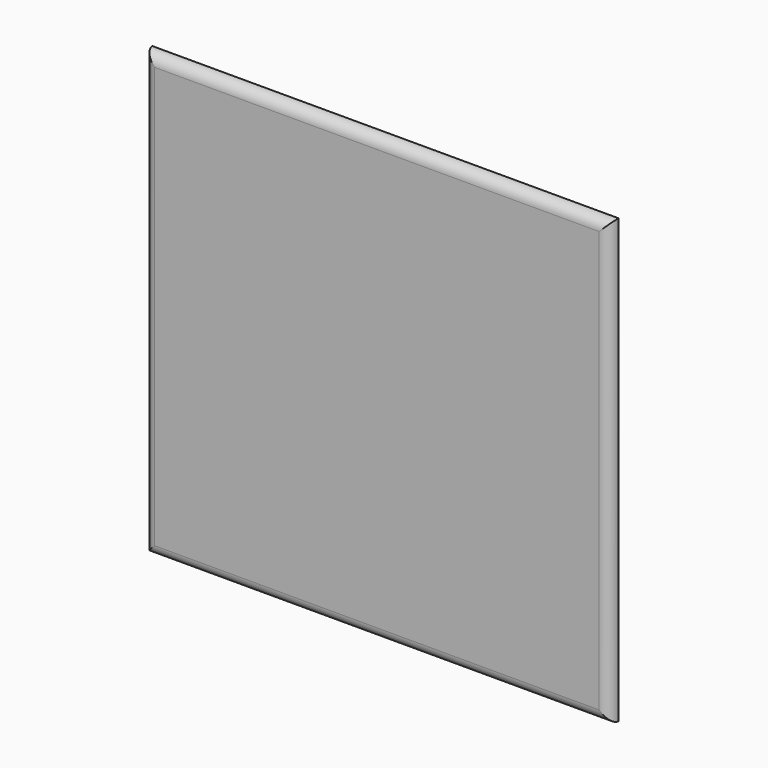
from build123d import *

# Parameters (mm, degrees)
F0_W     = 219.2782
F0_H     = 208.28
F1_DEPTH = 2.54
F2_R     = 5.07999


# Not quite as in the source:
# - a fillet or chamfer is up to 0.001 mm smaller than in the source, because OpenCascade refuses the exact size


with BuildPart() as f1:
    # F0 (on Front) → F1 (new body, symmetric)
    with BuildSketch(Plane.XZ):
        with Locations((26.8013083044, 9.9156468416)):
            Rectangle(F0_W, F0_H)
    extrude(amount=F1_DEPTH, both=True)

    # F2 (radius 5.08 in the source; OpenCascade refuses exactly that, so slightly less here)
    f2_edges = [f1.edges().sort_by_distance(p)[0] for p in [
        (26.801308, -2.54, 114.055647),
        (-82.837792, -2.54, 9.915647),
        (26.801308, -2.54, -94.224353),
        (136.440408, -2.54, 9.915647),
    ]]
    fillet(f2_edges, radius=F2_R)


solid = f1.part
